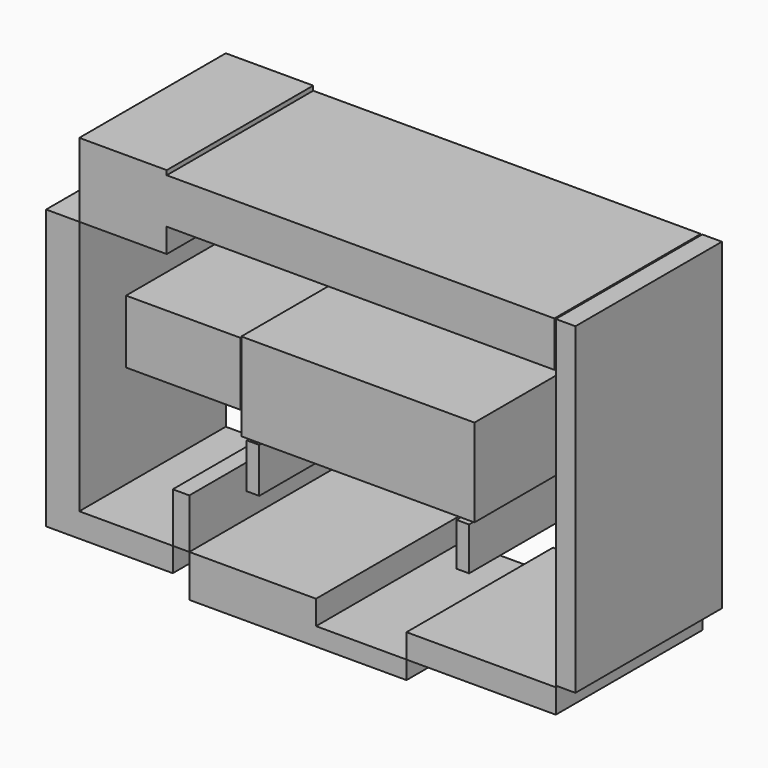
from build123d import *

# Parameters (mm, degrees)
F0_W     = 32.3380418122
F0_H     = 12.1889561415
F2_DEPTH = 25.4
F1_W     = 1.741277054
F1_H     = 6.2188543379
F3_DEPTH = 25.4
F1_W_2   = 1.7412863672
F1_H_2   = 5.9700999409
F4_W     = 15.8974092919
F4_H     = 8.7854117155
F5_DEPTH = 25.4
F4_W_2   = 20.7084715366
F4_H_2   = 3.3468240872
F4_W_3   = 12.5505886972
F4_H_3   = 2.5101173669
F4_W_4   = 33.2590593025
F4_H_4   = 6.275292486
F4_W_5   = 1.2550577521
F4_W_6   = 19.2442387342
F4_W_7   = 4.601882305
F4_H_5   = 35.3508265689
F4_W_8   = 2.3009395227
F4_H_6   = 6.9028222933
F4_W_9   = 2.7192905545
F4_H_7   = 17.1524714679
F4_H_8   = 27.6112947613


# Not quite as in the source:
# - a feature names something its author has since deleted; it is built from what else it names


with BuildPart() as f2:
    # F0 (on Front) → F2 (new body)
    with BuildSketch(Plane.XZ):
        with Locations((34.6703026444, 34.3791767955)):
            Rectangle(F0_W, F0_H)
    extrude(amount=F2_DEPTH)


with BuildPart() as f3:
    # F1 (on Front) → F3 (new body)
    with BuildSketch(Plane.XZ):
        with Locations((20.1181834564, 24.9265171587)):
            Rectangle(F1_W, F1_H)
    extrude(amount=F3_DEPTH)


with BuildPart() as f3b:
    # F1 (on Front) → F3, piece 2 (new body)
    with BuildSketch(Plane.XZ):
        with Locations((49.2224190384, 24.8021399602)):
            Rectangle(F1_W_2, F1_H_2)
    extrude(amount=F3_DEPTH)


with BuildPart() as f5:
    # F4 (on Front) → F5 (new body)
    with BuildSketch(Plane.XZ):
        with Locations((10.4588227114, 35.8737669885)):
            Rectangle(F4_W, F4_H)
    extrude(amount=F5_DEPTH)


with BuildPart() as f5b:
    # F4 (on Front) → F5, piece 2 (new body)
    with BuildSketch(Plane.XZ):
        with Locations((51.7711788416, 10.1450593211)):
            Rectangle(F4_W_2, F4_H_2)
    extrude(amount=F5_DEPTH)


with BuildPart() as f5c:
    # F4 (on Front) → F5, piece 3 (new body)
    with BuildSketch(Plane.XZ):
        Polygon((28.8663543761, 11.8184713647), (11.2955290824, 11.8184713647), (11.2955290824, 5.9615299106), (28.8663543761, 5.9615299106), (28.8663543761, 8.4716472775), align=None)
        with Locations((35.1416487247, 7.216588594)):
            Rectangle(F4_W_3, F4_H_3)
    extrude(amount=F5_DEPTH)


with BuildPart() as f5d:
    # F4 (on Front) → F5, piece 4 (new body)
    with BuildSketch(Plane.XZ):
        Polygon((-3.9743534289, 57.4189424515), (-3.9743534289, 47.1692979336), (8.1578837708, 47.1692979336), (8.1578837708, 50.5161210895), (8.1578837708, 56.7914135754), (8.1578837708, 57.4189424515), align=None)
        with Locations((24.787413422, 53.6537673324)):
            Rectangle(F4_W_4, F4_H_4)
        with Locations((42.0444719493, 53.6537673324)):
            Rectangle(F4_W_5, F4_H_4)
        with Locations((52.2941201925, 53.6537673324)):
            Rectangle(F4_W_6, F4_H_4)
    extrude(amount=F5_DEPTH)


with BuildPart() as f5e:
    # F4 (on Front) → F5, piece 5 (new body)
    with BuildSketch(Plane.XZ):
        Polygon((8.9945895597, 8.4716472775), (8.9945895597, 11.8184713647), (-3.9743534289, 11.8184713647), (-8.5762357339, 11.8184713647), (-8.5762357339, 8.4716472775), align=None)
        with Locations((-6.2752945814, 29.4938846491)):
            Rectangle(F4_W_7, F4_H_5)
    extrude(amount=F5_DEPTH)


with BuildPart() as f5f:
    # F4 (on Front) → F5, piece 6 (new body)
    with BuildSketch(Plane.XZ):
        with Locations((10.1450593211, 15.2698825113)):
            Rectangle(F4_W_8, F4_H_6)
    extrude(amount=F5_DEPTH)


with BuildPart() as f5g:
    # F4 (on Front) → F5, piece 7 (new body)
    with BuildSketch(Plane.XZ):
        with Locations((63.4850598872, 20.6038830802)):
            Rectangle(F4_W_9, F4_H_7)
        with Locations((63.4850598872, 42.9857661948)):
            Rectangle(F4_W_9, F4_H_8)
    extrude(amount=F5_DEPTH)


solid = Compound([f2.part, f3.part, f3b.part, f5.part, f5b.part, f5c.part, f5d.part, f5e.part, f5f.part, f5g.part])
